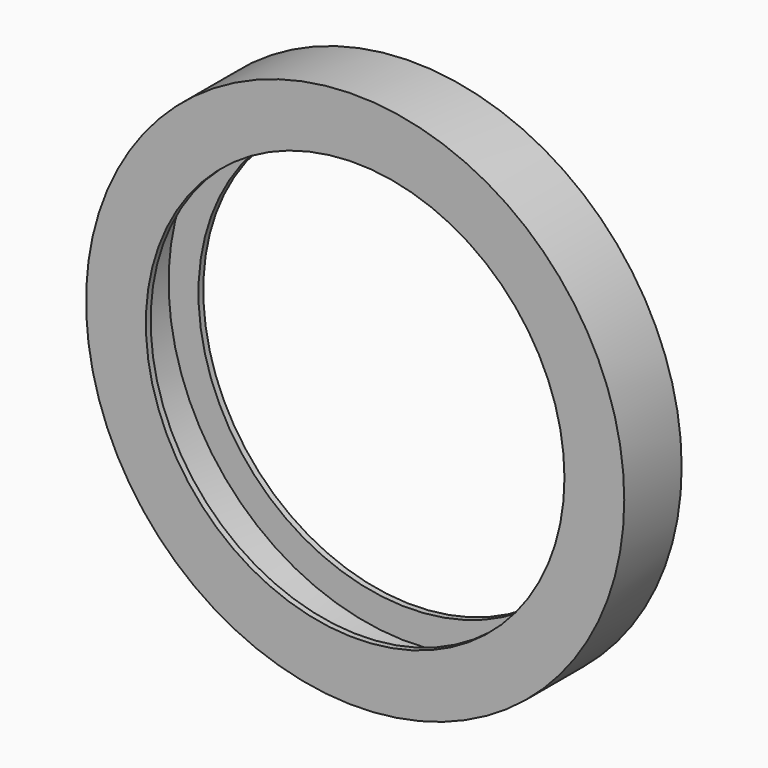
from build123d import *

# Parameters (mm, degrees)
F0_R     = 22.5
F0_R_2   = 20
F1_DEPTH = 3
F2_R     = 20
F2_R_2   = 17.5
F3_DEPTH = 0.5


# Not quite as in the source:
# - a pattern or mirror of a feature is missing from the dataset's text; its kind, count and spacing are read off the source's solid


with BuildPart() as f1:
    # F0 (on Front) → F1 (new body, symmetric)
    with BuildSketch(Plane.XZ):
        Circle(F0_R)
        Circle(F0_R_2, mode=Mode.SUBTRACT)
    extrude(amount=F1_DEPTH, both=True)

    # F2 (on face) → F3 (join)
    with BuildSketch(Plane.XZ.offset(3)):
        Circle(F2_R)
        Circle(F2_R_2, mode=Mode.SUBTRACT)
    f3 = extrude(amount=-F3_DEPTH)

    # F3_copies: F3 across plane
    add(f3.mirror(Plane.ZX))


solid = f1.part
